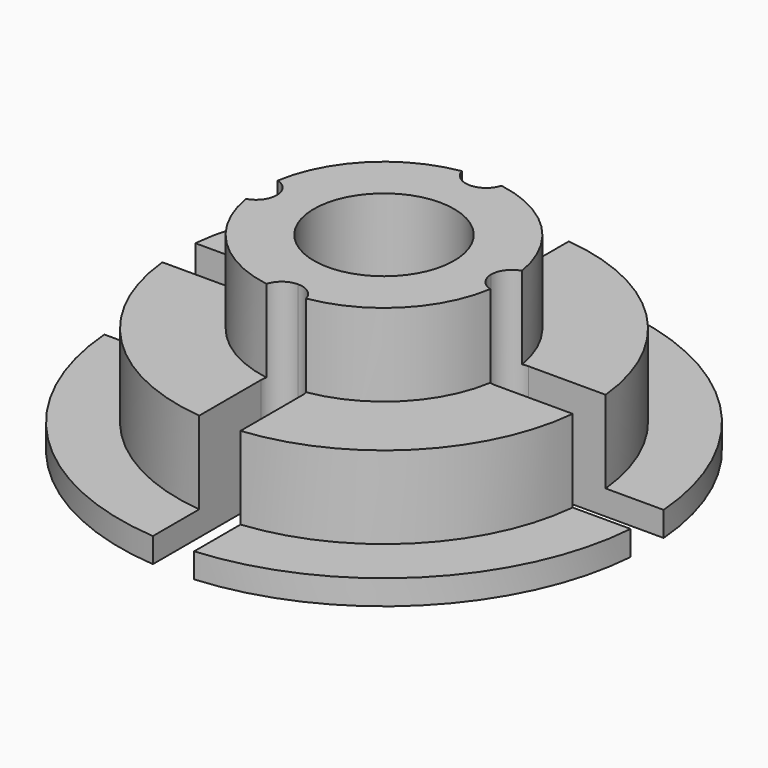
from build123d import *

# Parameters (mm, degrees)
F3_DEPTH = 23.001
F4_R     = 2.5
F4_R_2   = 2.49999


# Not quite as in the source:
# - a fillet or chamfer is up to 0.001 mm smaller than in the source, because OpenCascade refuses the exact size


with BuildPart() as f1:
    # F0 (on Right) → F1 (revolve)
    with BuildSketch(Plane.YZ):
        Polygon((8.5, 23), (8.5, 0), (32, 0), (32, 3), (25, 3), (25, 13), (15, 13), (15, 23), align=None)
    revolve(axis=Axis((0, 0, 31.7647196352), (0, 0, 1)))

    # F2 (on face) → F3 (cut, through all)
    with BuildSketch(Plane(origin=(0, 0, 0), x_dir=(1, 0, 0), z_dir=(0, 0, -1))):
        with BuildLine():
            Line((-2.5, 13), (2.5, 13))
            Line((2.5, 13), (2.5, 31.9021942819))
            ThreePointArc((2.5, 31.9021942819), (0, 32), (-2.5, 31.9021942819))
            Line((-2.5, 31.9021942819), (-2.5, 13))
        make_face()
        with BuildLine():
            ThreePointArc((32, 0), (31.9755392216, 1.2509562301), (31.9021942819, 2.5))
            Line((31.9021942819, 2.5), (13, 2.5))
            Line((13, 2.5), (13, -2.5))
            Line((13, -2.5), (31.9021942819, -2.5))
            ThreePointArc((31.9021942819, -2.5), (31.9755392216, -1.2509562301), (32, 0))
        make_face()
        with BuildLine():
            Line((-2.5, -13), (-2.5, -31.9021942819))
            ThreePointArc((-2.5, -31.9021942819), (0, -32), (2.5, -31.9021942819))
            Line((2.5, -31.9021942819), (2.5, -13))
            Line((2.5, -13), (-2.5, -13))
        make_face()
        with BuildLine():
            Line((-13, 2.5), (-31.9021942819, 2.5))
            ThreePointArc((-31.9021942819, 2.5), (-32, 0), (-31.9021942819, -2.5))
            Line((-31.9021942819, -2.5), (-13, -2.5))
            Line((-13, -2.5), (-13, 2.5))
        make_face()
    extrude(amount=-F3_DEPTH, mode=Mode.SUBTRACT)

    # F4 (call 1 of 8: OpenCascade refuses the feature's edges together)
    f4_edges = [f1.edges().sort_by_distance(p)[0] for p in [
        (-2.5, -13, 11.5),
    ]]
    fillet(f4_edges, radius=F4_R)

    # F4#2 (call 2 of 8) (radius 2.5 in the source; OpenCascade refuses exactly that, so slightly less here)
    f4_2_edges = [f1.edges().sort_by_distance(p)[0] for p in [
        (2.5, -13, 11.5),
    ]]
    fillet(f4_2_edges, radius=F4_R_2)

    # F4#3 (call 3 of 8)
    f4_3_edges = [f1.edges().sort_by_distance(p)[0] for p in [
        (13, -2.5, 11.5),
    ]]
    fillet(f4_3_edges, radius=F4_R)

    # F4#4 (call 4 of 8) (radius 2.5 in the source; OpenCascade refuses exactly that, so slightly less here)
    f4_4_edges = [f1.edges().sort_by_distance(p)[0] for p in [
        (13, 2.5, 11.5),
    ]]
    fillet(f4_4_edges, radius=F4_R_2)

    # F4#5 (call 5 of 8)
    f4_5_edges = [f1.edges().sort_by_distance(p)[0] for p in [
        (-2.5, 13, 11.5),
    ]]
    fillet(f4_5_edges, radius=F4_R)

    # F4#6 (call 6 of 8) (radius 2.5 in the source; OpenCascade refuses exactly that, so slightly less here)
    f4_6_edges = [f1.edges().sort_by_distance(p)[0] for p in [
        (2.5, 13, 11.5),
    ]]
    fillet(f4_6_edges, radius=F4_R_2)

    # F4#7 (call 7 of 8)
    f4_7_edges = [f1.edges().sort_by_distance(p)[0] for p in [
        (-13, 2.5, 11.5),
    ]]
    fillet(f4_7_edges, radius=F4_R)

    # F4#8 (call 8 of 8) (radius 2.5 in the source; OpenCascade refuses exactly that, so slightly less here)
    f4_8_edges = [f1.edges().sort_by_distance(p)[0] for p in [
        (-13, -2.5, 11.5),
    ]]
    fillet(f4_8_edges, radius=F4_R_2)


solid = f1.part
